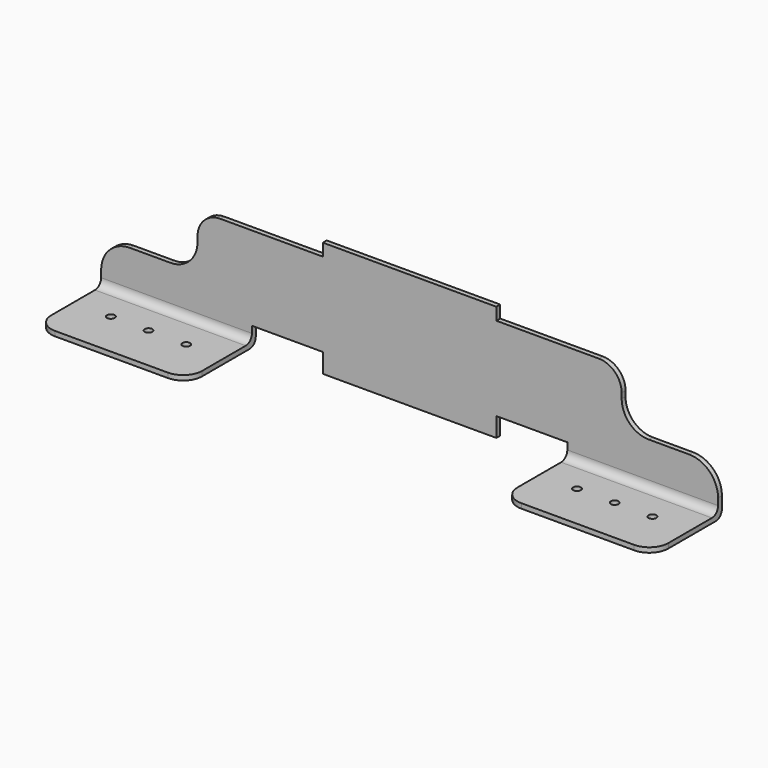
from build123d import *

# Parameters (mm, degrees)
F0_W     = 63.5
F0_H     = 28.575
F0_W_2   = 46.736
F0_H_2   = 27.6352
F0_W_3   = 57.15
F0_H_3   = 8.128
F1_DEPTH = 3.175
F0_H_4   = 3.175
F0_W_4   = 35.814
F2_DEPTH = 56.642
F3_R     = 18.991869689
F4_R     = 17.8311640925
F5_R     = 14.9730007981
F6_R     = 5.08
F7_R     = 12.4823532344
F9_D     = 5.08
F9_DEPTH = 25.4
F9_TIP   = 1.5261859723


# Not quite as in the source:
# - a feature names something its author has since deleted; it is built from what else it names


with BuildPart() as f1:
    # F0 (on Front) → F1 (new body)
    with BuildSketch(Plane.XZ):
        with Locations((-171.45, 17.4625)):
            Rectangle(F0_W, F0_H)
        Polygon((-57.15, 0), (0, 0), (0, 40.3352), (-57.15, 40.3352), (-57.15, 12.7), align=None)
        with Locations((-80.518, 26.5176)):
            Rectangle(F0_W_2, F0_H_2)
        with Locations((-80.518, 54.1528)):
            Rectangle(F0_W_2, F0_H_2)
        Polygon((-103.886, 3.175), (-103.886, 12.7), (-103.886, 40.3352), (-103.886, 67.9704), (-139.7, 67.9704), (-139.7, 31.75), (-139.7, 3.175), align=None)
        with Locations((-28.575, 54.1528)):
            Rectangle(F0_W_3, F0_H_2)
        with Locations((-28.575, 72.0344)):
            Rectangle(F0_W_3, F0_H_3)
    extrude(amount=F1_DEPTH)

    # F0 (on Front) → F2 (join)
    with BuildSketch(Plane.XZ):
        with Locations((-171.45, 1.5875)):
            Rectangle(F0_W, F0_H_4)
        with Locations((-121.793, 1.5875)):
            Rectangle(F0_W_4, F0_H_4)
    extrude(amount=F2_DEPTH)

    # F3
    f3_edges = [f1.edges().sort_by_distance(p)[0] for p in [
        (-203.2, -1.5875, 31.75),
    ]]
    fillet(f3_edges, radius=F3_R)

    # F4
    f4_edges = [f1.edges().sort_by_distance(p)[0] for p in [
        (-139.7, -1.5875, 31.75),
    ]]
    fillet(f4_edges, radius=F4_R)

    # F5
    f5_edges = [f1.edges().sort_by_distance(p)[0] for p in [
        (-139.7, -1.5875, 67.9704),
    ]]
    fillet(f5_edges, radius=F5_R)

    # F6
    f6_edges = [f1.edges().sort_by_distance(p)[0] for p in [
        (-153.543, 0, 0),
        (-153.543, -3.175, 3.175),
    ]]
    fillet(f6_edges, radius=F6_R)

    # F7
    f7_edges = [f1.edges().sort_by_distance(p)[0] for p in [
        (-103.886, -56.642, 1.5875),
        (-203.2, -56.642, 1.5875),
    ]]
    fillet(f7_edges, radius=F7_R)

    # F9
    with Locations(Plane.XY.offset(3.175)):
        with Locations((-153.543, -26.2073233828), (-128.7145, -26.2073233828), (-178.3715, -26.2073233828)):
            Hole(F9_D / 2, depth=F9_DEPTH)
            with Locations((0, 0, -(F9_DEPTH + F9_TIP / 2))):  # 118° drill point
                Cone(0, F9_D / 2, F9_TIP, mode=Mode.SUBTRACT)

    # F10: F1 across face


with BuildPart() as f1_1:
    add(f1.part)
    add(f1.part.mirror(Plane(origin=(0, -1.5875, 38.0492), x_dir=(0, 1, 0), z_dir=(1, 0, 0))))


solid = f1_1.part
